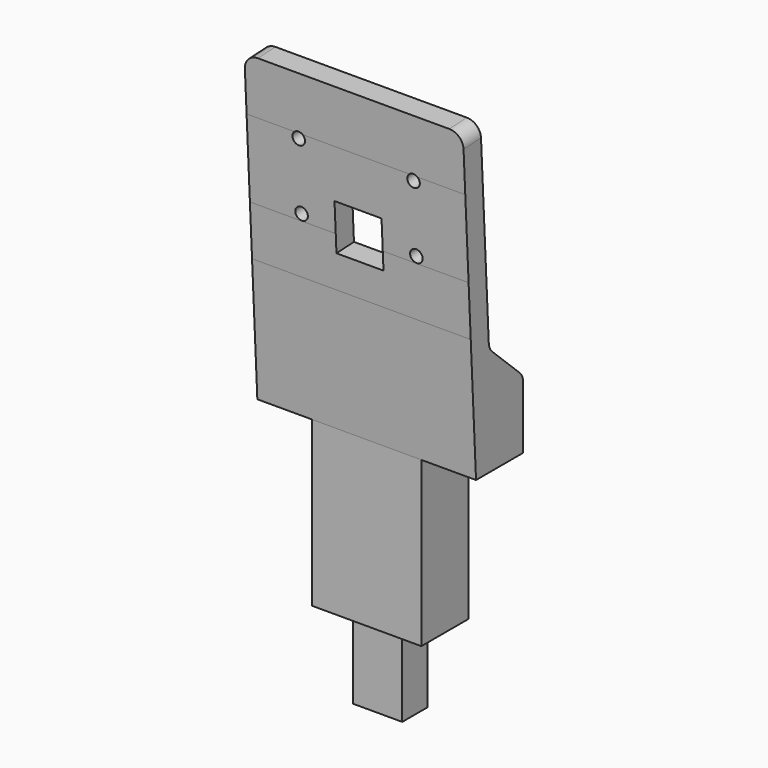
from build123d import *

# Parameters (mm, degrees)
F0_W          = 20
F0_H          = 10.77
F1_DEPTH      = 10
F1_DEPTH_BACK = 20
F3_DEPTH      = 30
F3_DEPTH_BACK = 10
F4_DEPTH      = 10
F5_R          = 1.15
F6_DEPTH      = 25
F7_W          = 9
F7_H          = 5.77
F8_DEPTH      = 15
F9_R          = 2.5
F10_R         = 2.5


with BuildPart() as f1:
    # F0 (on Top) → F1 (new body, two sides)
    with BuildSketch(Plane.XY) as f1_sk:
        with Locations((4.4768884756, -0.816908665)):
            Rectangle(F0_W, F0_H)
    extrude(amount=F1_DEPTH)
    extrude(f1_sk.sketch, amount=-F1_DEPTH_BACK)

    # F2 (on face) → F3 (join, two sides)
    with BuildSketch(Plane(origin=(-5.5231115244, 0, 0), x_dir=(0, -1, 0), z_dir=(-1, 0, 0))) as f3_sk:
        Polygon((7.9035344876, 42.4689549124), (8.6624058531, 56.9490831664), (4.6678877141, 57.1584269913), (3.2377782985, 29.8703137532), (-4.568091335, 22.4698111415), (-4.568091335, 10), (6.201908665, 10), (7.4136699372, 33.1217824671), align=None)
    extrude(amount=-F3_DEPTH)
    extrude(f3_sk.sketch, amount=F3_DEPTH_BACK)

    # F4 (add): a face of the model
    f4_faces = [f1.faces().sort_by_distance(p)[0] for p in [
        (4.4768884756, -6.6651467836, 57.0537550789),
    ]]
    extrude(f4_faces, amount=F4_DEPTH)

    # F5 (on face) → F6 (cut)
    with BuildSketch(Plane(origin=(0, -5.6622789964, -0.2967474679), x_dir=(1, 0, 0), z_dir=(0, -0.9986295348, -0.0523359562))):
        Polygon((8.7768884756, 48.1932846266), (4.4768884756, 48.1932846266), (0.1768884756, 48.1932846266), (0.1768884756, 39.5932846266), (8.7768884756, 39.5932846266), align=None)
        with Locations((14.9768884756, 56.4432846266)):
            Circle(F5_R)
        with Locations((14.9768884756, 44.0432846266)):
            Circle(F5_R)
        with Locations((-6.0231115244, 44.0432846266)):
            Circle(F5_R)
        with Locations((-6.0231115244, 56.4432846266)):
            Circle(F5_R)
    extrude(amount=-F6_DEPTH, mode=Mode.SUBTRACT)

    # F7 (on face) → F8 (join)
    with BuildSketch(Plane(origin=(0, 0, -20), x_dir=(1, 0, 0), z_dir=(0, 0, -1))):
        with Locations((4.4768884756, 0.816908665)):
            Rectangle(F7_W, F7_H)
    extrude(amount=F8_DEPTH)

    # F9
    f9_edges = [f1.edges().sort_by_distance(p)[0] for p in [
        (-15.523112, -7.188506, 67.04005),
        (24.476888, -7.188506, 67.04005),
    ]]
    fillet(f9_edges, radius=F9_R)

    # F10
    f10_edges = [f1.edges().sort_by_distance(p)[0] for p in [
        (4.476888, -3.237778, 29.870314),
        (4.476888, 4.568091, 22.469811),
    ]]
    fillet(f10_edges, radius=F10_R)


solid = f1.part
